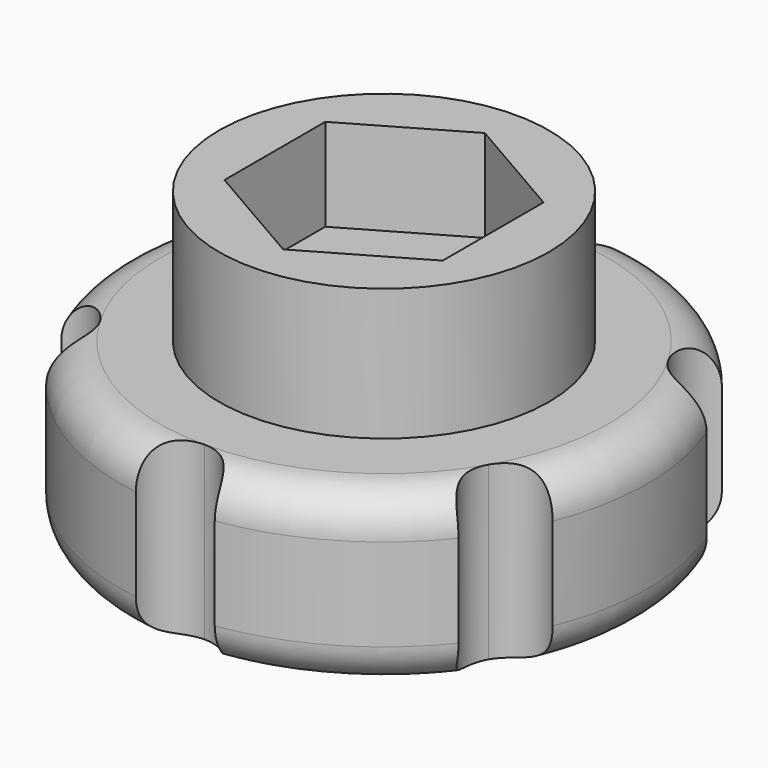
from build123d import *

# Parameters (mm, degrees)
F0_R     = 20
F1_DEPTH = 13
F2_R     = 12.5
F3_DEPTH = 10
F4_R     = 3
F6_DEPTH = 7
F8_DEPTH = 25


with BuildPart() as f1:
    # F0 (on Top) → F1 (new body)
    with BuildSketch(Plane.XY):
        Circle(F0_R)
    extrude(amount=F1_DEPTH)

    # F2 (on face) → F3 (join)
    with BuildSketch(Plane.XY.offset(13)):
        Circle(F2_R)
    extrude(amount=F3_DEPTH)

    # F4
    f4_edges = [f1.edges().sort_by_distance(p)[0] for p in [
        (-20, 0, 13),
        (-20, 0, 0),
    ]]
    fillet(f4_edges, radius=F4_R)

    # F5 (on face) → F6 (cut)
    with BuildSketch(Plane.XY.offset(23)):
        Polygon((8.2705426061, 4.775), (0, 9.55), (-8.2705426061, 4.775), (-8.2705426061, -4.775), (0, -9.55), (8.2705426061, -4.775), align=None)
    extrude(amount=-F6_DEPTH, mode=Mode.SUBTRACT)

    # F7 (on face) → F8 (cut)
    with BuildSketch(Plane(origin=(0, 0, 0), x_dir=(1, 0, 0), z_dir=(0, 0, -1))):
        with BuildLine():
            ThreePointArc((14.7224318372, 8.5000000471), (16.435854573, 7.1334012872), (18.6214276605, 7.2967411826))
            ThreePointArc((18.6214276605, 7.2967411826), (17.3205080757, 10), (15.6298770592, 12.4782588174))
            ThreePointArc((15.6298770592, 12.4782588174), (14.3956340287, 10.6671670025), (14.7224318372, 8.5000000471))
        make_face()
        with BuildLine():
            ThreePointArc((20.3205080757, -10), (19.8604646456, -8.4035600159), (18.6214276605, -7.2967411826))
            ThreePointArc((18.6214276605, -7.2967411826), (17.3205080757, -10), (15.6298770592, -12.4782588174))
            ThreePointArc((15.6298770592, -12.4782588174), (18.7219549977, -12.6525358668), (20.3205080757, -10))
        make_face()
        with BuildLine():
            ThreePointArc((15.6298770592, -12.4782588174), (17.3205080757, -10), (18.6214276605, -7.2967411826))
            ThreePointArc((18.6214276605, -7.2967411826), (16.435854533, -7.1334012995), (14.7224317953, -8.5000001196))
            ThreePointArc((14.7224317953, -8.5000001196), (14.395634038, -10.6671670433), (15.6298770592, -12.4782588174))
        make_face()
        with BuildLine():
            ThreePointArc((-1.46e-08, 17), (2.040220571, 17.8005682502), (2.9915506013, 19.775))
            ThreePointArc((2.9915506013, 19.775), (0, 20), (-2.9915506013, 19.775))
            ThreePointArc((-2.9915506013, 19.775), (-2.0402205817, 17.8005682602), (-1.46e-08, 17))
        make_face()
        with BuildLine():
            ThreePointArc((-2.9915506013, 19.775), (0, 20), (2.9915506013, 19.775))
            ThreePointArc((2.9915506013, 19.775), (2.9978869061, 19.8874207031), (3, 20))
            ThreePointArc((3, 20), (-0.1125792969, 22.9978869061), (-2.9915506013, 19.775))
        make_face()
        with BuildLine():
            ThreePointArc((3, -20), (2.9978869061, -19.8874207031), (2.9915506013, -19.775))
            ThreePointArc((2.9915506013, -19.775), (0, -20), (-2.9915506013, -19.775))
            ThreePointArc((-2.9915506013, -19.775), (-0.1125792969, -22.9978869061), (3, -20))
        make_face()
        with BuildLine():
            ThreePointArc((-2.9915506013, -19.775), (0, -20), (2.9915506013, -19.775))
            ThreePointArc((2.9915506013, -19.775), (2.0402205635, -17.8005682433), (-3.5e-08, -17))
            ThreePointArc((-3.5e-08, -17), (-2.0402205891, -17.8005682671), (-2.9915506013, -19.775))
        make_face()
        with BuildLine():
            ThreePointArc((-18.6214276605, 7.2967411826), (-16.4358546167, 7.1334012737), (-14.7224318829, 8.4999999678))
            ThreePointArc((-14.7224318829, 8.4999999678), (-14.4227306016, 9.2235428467), (-14.3205080757, 10))
            ThreePointArc((-14.3205080757, 10), (-14.6679722089, 11.401446922), (-15.6298770592, 12.4782588174))
            ThreePointArc((-15.6298770592, 12.4782588174), (-17.3205080757, 10), (-18.6214276605, 7.2967411826))
        make_face()
        with BuildLine():
            ThreePointArc((-14.3205080757, -10), (-14.4227305909, -9.2235428867), (-14.7224318416, -8.5000000394))
            ThreePointArc((-14.7224318416, -8.5000000394), (-16.4358545772, -7.1334012859), (-18.6214276605, -7.2967411826))
            ThreePointArc((-18.6214276605, -7.2967411826), (-17.3205080757, -10), (-15.6298770592, -12.4782588174))
            ThreePointArc((-15.6298770592, -12.4782588174), (-14.6679722089, -11.401446922), (-14.3205080757, -10))
        make_face()
        with BuildLine():
            ThreePointArc((-18.6214276605, 7.2967411826), (-17.3205080757, 10), (-15.6298770592, 12.4782588174))
            ThreePointArc((-15.6298770592, 12.4782588174), (-19.918584287, 11.5), (-18.6214276605, 7.2967411826))
        make_face()
        with BuildLine():
            ThreePointArc((-18.6214276605, -7.2967411826), (-19.918584287, -11.5), (-15.6298770592, -12.4782588174))
            ThreePointArc((-15.6298770592, -12.4782588174), (-17.3205080757, -10), (-18.6214276605, -7.2967411826))
        make_face()
    extrude(amount=-F8_DEPTH, mode=Mode.SUBTRACT)


solid = f1.part
